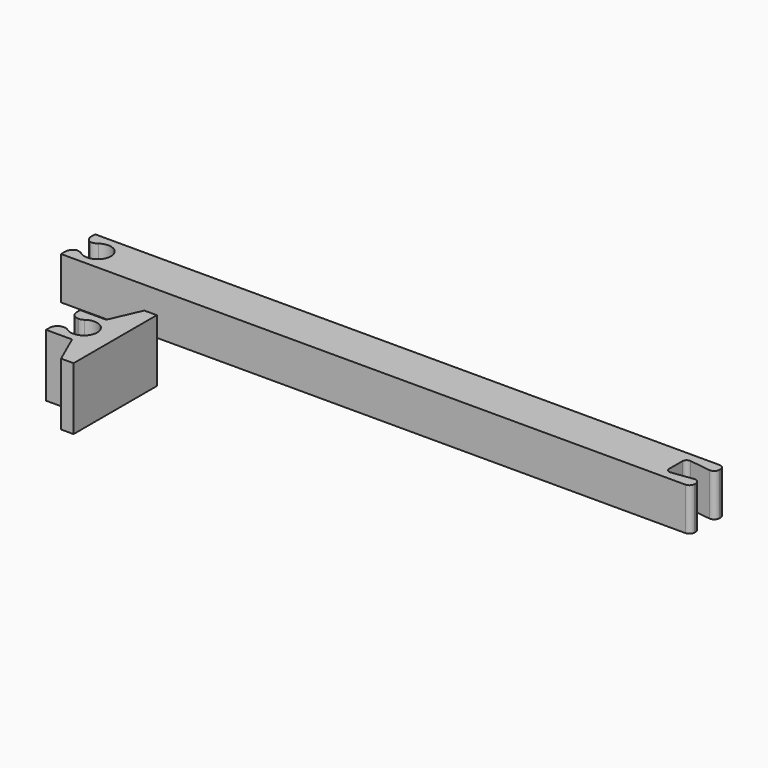
from build123d import *

# Parameters (mm, degrees)
F1_DEPTH    = 8.2
F2_R        = 2
F3_T1_DEPTH = 15.4242863712
F4_R        = 2
F5_T1_DEPTH = 15.4242863712
F6_R        = 1
F7_R        = 1
F8_R        = 0.8
F9_R        = 0.8
F10_W       = 2.4
F10_H       = 5.9
F10_H_2     = 8.2
F11_DEPTH   = 12
F12_R       = 1.5
F13_R       = 1.5


# Not quite as in the source:
# - a fillet or chamfer that OpenCascade refuses, or shapes differently, is made with other operations: its cross-section is extruded or revolved along the edge and cut away or added


with BuildPart() as f1:
    # F0 (on Top) → F1 (new body)
    with BuildSketch(Plane.XY):
        with BuildLine():
            Line((70.2436813011, -1.2552053894), (-50.7563186989, -1.2552053894))
            Line((-50.7563186989, -1.2552053894), (-50.7563186989, -3.6802053894))
            Line((-50.7563186989, -3.6802053894), (-48.8993186989, -3.6802053894))
            ThreePointArc((-48.8993186989, -3.6802053894), (-46.0822916792, -2.9671673746), (-44.4265927694, -5.3552053894))
            ThreePointArc((-44.4265927694, -5.3552053894), (-46.0822916792, -7.7432434042), (-48.8993186989, -7.0302053894))
            Line((-48.8993186989, -7.0302053894), (-50.7563186989, -7.0302053894))
            Line((-50.7563186989, -7.0302053894), (-50.7563186989, -9.4552053894))
            Line((-50.7563186989, -9.4552053894), (70.2436813011, -9.4552053894))
            Line((70.2436813011, -9.4552053894), (70.2436813011, -7.0552053894))
            Line((70.2436813011, -7.0552053894), (64.1436813011, -7.8552053894))
            Line((64.1436813011, -7.8552053894), (64.1436813011, -2.8552053894))
            Line((64.1436813011, -2.8552053894), (70.2436813011, -3.6552053894))
            Line((70.2436813011, -3.6552053894), (70.2436813011, -1.2552053894))
        make_face()
    extrude(amount=F1_DEPTH)

    # F2
    f2_edges = [f1.edges().sort_by_distance(p)[0] for p in [
        (-48.899319, -7.030205, 4.1),
    ]]
    fillet(f2_edges, radius=F2_R)

    # F3: fillet of radius 1.5 on 1 edges, made by hand

    # F3_s2 → F3_t1 (cut)
    with BuildSketch(Plane.XY.offset(-3.6121431856)):
        with BuildLine():
            ThreePointArc((-49.6592919698, -7.0302053894), (-50.450985997, -7.5679959369), (-50.7563186989, -8.4750626637))
            Line((-50.7563186989, -8.4750626637), (-50.7863186989, -8.4750626637))
            Line((-50.7863186989, -8.4750626637), (-50.7863186989, -7.0302053894))
            Line((-50.7863186989, -7.0302053894), (-50.7563186989, -7.0002053894))
            ThreePointArc((-50.7563186989, -7.0002053894), (-50.2078053343, -7.0002053894), (-49.6673514352, -7.0013082439))
            Line((-49.6673514352, -7.0013082439), (-49.6592919698, -7.0302053894))
        make_face()
    extrude(amount=F3_T1_DEPTH, mode=Mode.SUBTRACT)

    # F4
    f4_edges = [f1.edges().sort_by_distance(p)[0] for p in [
        (-48.899319, -3.680205, 4.1),
    ]]
    fillet(f4_edges, radius=F4_R)

    # F5: fillet of radius 1.5 on 1 edges, made by hand

    # F5_s2 → F5_t1 (cut)
    with BuildSketch(Plane.XY.offset(-3.6121431856)):
        with BuildLine():
            ThreePointArc((-49.6592919698, -3.6802053894), (-50.450985997, -3.142414842), (-50.7563186989, -2.2353481152))
            Line((-50.7563186989, -2.2353481152), (-50.7863186989, -2.2353481152))
            Line((-50.7863186989, -2.2353481152), (-50.7863186989, -3.6802053894))
            Line((-50.7863186989, -3.6802053894), (-50.7563186989, -3.7102053894))
            ThreePointArc((-50.7563186989, -3.7102053894), (-50.2078053343, -3.7102053894), (-49.6673514352, -3.7091025349))
            Line((-49.6673514352, -3.7091025349), (-49.6592919698, -3.6802053894))
        make_face()
    extrude(amount=F5_T1_DEPTH, mode=Mode.SUBTRACT)

    # F6
    f6_edges = [f1.edges().sort_by_distance(p)[0] for p in [
        (70.243681, -3.655205, 4.1),
        (70.243681, -7.055205, 4.1),
    ]]
    fillet(f6_edges, radius=F6_R)

    # F7
    f7_edges = [f1.edges().sort_by_distance(p)[0] for p in [
        (70.243681, -1.255205, 4.1),
        (70.243681, -9.455205, 4.1),
    ]]
    fillet(f7_edges, radius=F7_R)

    # F8
    f8_edges = [f1.edges().sort_by_distance(p)[0] for p in [
        (64.143681, -2.855205, 4.1),
    ]]
    fillet(f8_edges, radius=F8_R)

    # F9
    f9_edges = [f1.edges().sort_by_distance(p)[0] for p in [
        (64.143681, -7.855205, 4.1),
    ]]
    fillet(f9_edges, radius=F9_R)


with BuildPart() as f11:
    # F10 (on Top) → F11 (new body)
    with BuildSketch(Plane.XY):
        with BuildLine():
            Line((-27.546004492, -27.6037355185), (-32.546004492, -27.6037355185))
            Line((-32.546004492, -27.6037355185), (-32.546004492, -29.9537355185))
            Line((-32.546004492, -29.9537355185), (-30.4007281911, -29.9537355185))
            ThreePointArc((-30.4007281911, -29.9537355185), (-27.6044752659, -29.3339206066), (-25.996004492, -31.7037355185))
            ThreePointArc((-25.996004492, -31.7037355185), (-27.6044752659, -34.0735504303), (-30.4007281911, -33.4537355185))
            Line((-30.4007281911, -33.4537355185), (-32.546004492, -33.4537355185))
            Line((-32.546004492, -33.4537355185), (-32.546004492, -35.8037355185))
            Line((-32.546004492, -35.8037355185), (-27.546004492, -35.8037355185))
            Line((-27.546004492, -35.8037355185), (-24.946004492, -35.8037355185))
            Line((-24.946004492, -35.8037355185), (-24.946004492, -27.6037355185))
            Line((-24.946004492, -27.6037355185), (-27.546004492, -27.6037355185))
        make_face()
        Polygon((-24.946004492, -21.7037355185), (-27.546004492, -27.6037355185), (-24.946004492, -27.6037355185), align=None)
        with Locations((-23.746004492, -24.6537355185)):
            Rectangle(F10_W, F10_H)
        with Locations((-23.746004492, -31.7037355185)):
            Rectangle(F10_W, F10_H_2)
        with Locations((-23.746004492, -38.7537355185)):
            Rectangle(F10_W, F10_H)
        Polygon((-24.946004492, -41.7037355185), (-24.946004492, -35.8037355185), (-27.546004492, -35.8037355185), align=None)
    extrude(amount=F11_DEPTH)

    # F12
    f12_edges = [f11.edges().sort_by_distance(p)[0] for p in [
        (-32.546004, -33.453736, 6),
        (-32.546004, -29.953736, 6),
    ]]
    fillet(f12_edges, radius=F12_R)

    # F13
    f13_edges = [f11.edges().sort_by_distance(p)[0] for p in [
        (-30.400728, -29.953736, 6),
        (-30.400728, -33.453736, 6),
    ]]
    fillet(f13_edges, radius=F13_R)


solid = Compound([f1.part, f11.part])
